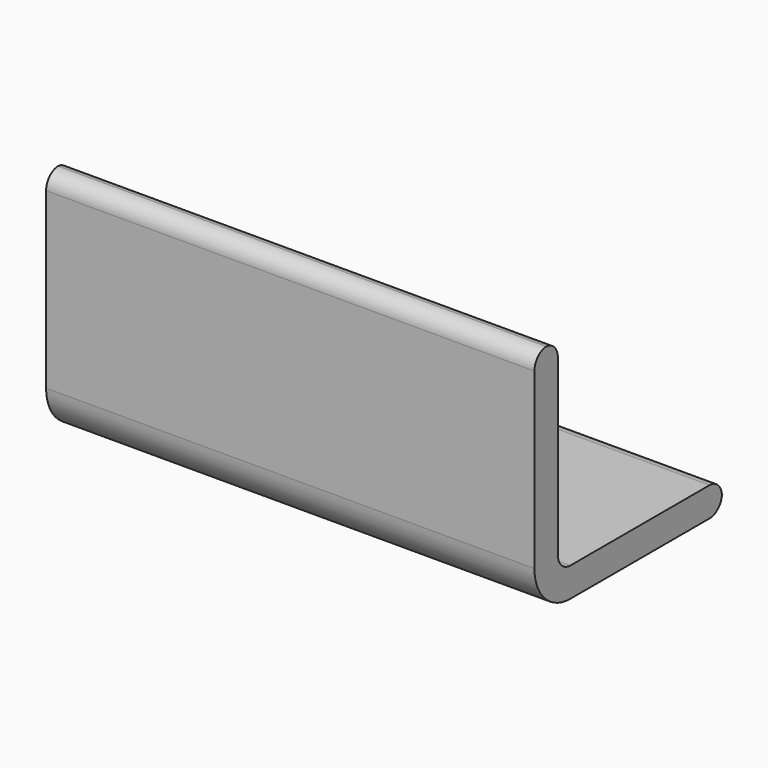
from build123d import *

# Parameters (mm, degrees)
F1_DEPTH    = 79.375
F2_T1_DEPTH = 79.375
F2_T3_DEPTH = 92.075
F3_R        = 7.3025


# Not quite as in the source:
# - a fillet or chamfer that OpenCascade refuses, or shapes differently, is made with other operations: its cross-section is extruded or revolved along the edge and cut away or added


with BuildPart() as f1:
    # F0 (on Right) → F1 (new body)
    with BuildSketch(Plane.YZ):
        Polygon((0, 38.1), (0, 0), (38.1, 0), (38.1, 4.7625), (4.7625, 4.7625), (4.7625, 38.1), align=None)
    extrude(amount=F1_DEPTH)

    # F2: fillet of radius 2.54 on 5 edges, made by hand

    # F2_s2 → F2_t1 (join)
    with BuildSketch(Plane.YZ):
        with BuildLine():
            ThreePointArc((7.3025, 4.7625), (5.5064487758, 5.5064487758), (4.7625, 7.3025))
            Line((4.7625, 7.3025), (4.7625, 4.7625))
            Line((4.7625, 4.7625), (7.3025, 4.7625))
        make_face()
    extrude(amount=F2_T1_DEPTH)

    # F2_s4 → F2_t3 (cut)
    with BuildSketch(Plane.YZ.offset(-6.35)):
        with BuildLine():
            ThreePointArc((2.2225, 38.1), (4.0185512242, 37.3560512242), (4.7625, 35.56))
            Line((4.7625, 35.56), (4.7625, 38.1))
            Line((4.7625, 38.1), (2.2225, 38.1))
        make_face()
        with BuildLine():
            ThreePointArc((0, 35.56), (0.7439487758, 37.3560512242), (2.54, 38.1))
            Line((2.54, 38.1), (0, 38.1))
            Line((0, 38.1), (0, 35.56))
        make_face()
        with BuildLine():
            ThreePointArc((38.1, 2.2225), (37.3560512242, 4.0185512242), (35.56, 4.7625))
            Line((35.56, 4.7625), (38.1, 4.7625))
            Line((38.1, 4.7625), (38.1, 2.2225))
        make_face()
        with BuildLine():
            ThreePointArc((35.56, 0), (37.3560512242, 0.7439487758), (38.1, 2.54))
            Line((38.1, 2.54), (38.1, 0))
            Line((38.1, 0), (35.56, 0))
        make_face()
    extrude(amount=F2_T3_DEPTH, mode=Mode.SUBTRACT)

    # F3
    f3_edges = [f1.edges().sort_by_distance(p)[0] for p in [
        (39.6875, 0, 0),
    ]]
    fillet(f3_edges, radius=F3_R)


solid = f1.part
